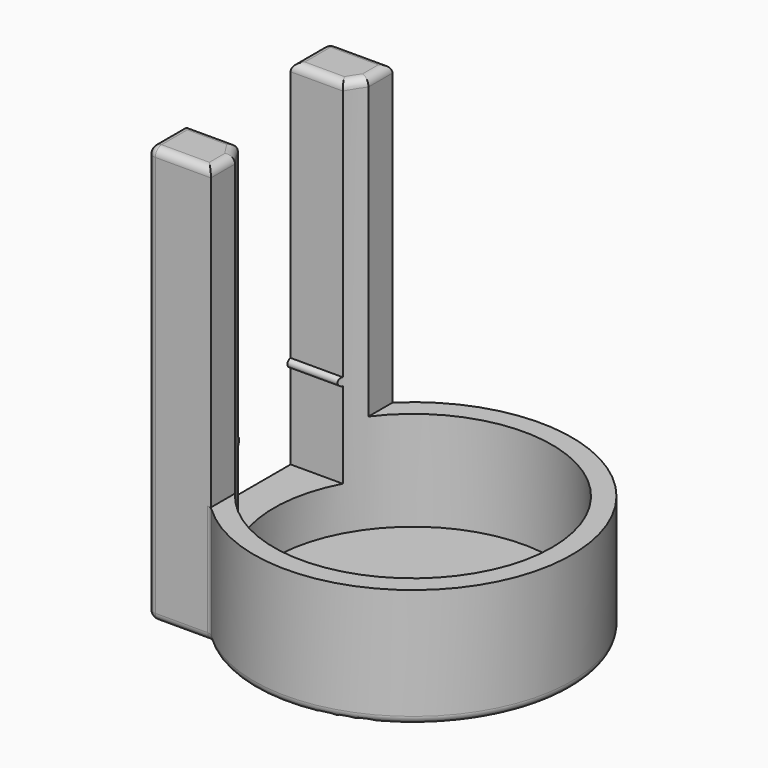
from build123d import *

# Parameters (mm, degrees)
F0_R      = 20
F1_DEPTH  = 50
F2_DEPTH  = 2.5
F4_W      = 40
F4_H      = 50
F5_DEPTH  = 25
F6_W      = 8
F6_H      = 28.5657137142
F7_DEPTH  = 2.5
F8_DEPTH  = 50
F3_R      = 17.5
F9_DEPTH  = 50
F11_DEPTH = 25
F12_R     = 1


with BuildPart() as f1:
    # F0 (on Top) → F1 (new body)
    with BuildSketch(Plane.XY):
        Circle(F0_R)
    extrude(amount=F1_DEPTH)

    # F2 (add): a face of the model
    f2_faces = [f1.faces().sort_by_distance(p)[0] for p in [
        (0, 0, 0),
    ]]
    extrude(f2_faces, amount=F2_DEPTH)

    # F4 (on Front) → F5 (cut, symmetric)
    with BuildSketch(Plane.XZ):
        with Locations((6, 37.5)):
            Rectangle(F4_W, F4_H)
    extrude(amount=F5_DEPTH, both=True, mode=Mode.SUBTRACT)

    # F6 (on Top) → F7 (join)
    with BuildSketch(Plane.XY):
        with Locations((-18, 0)):
            Rectangle(F6_W, F6_H)
    extrude(amount=-F7_DEPTH)

    # F6 (on Top) → F8 (join)
    with BuildSketch(Plane.XY):
        with Locations((-18, 0)):
            Rectangle(F6_W, F6_H)
    extrude(amount=F8_DEPTH)

    # F3 (on Top) → F9 (cut)
    with BuildSketch(Plane.XY):
        Circle(F3_R)
    extrude(amount=F9_DEPTH, mode=Mode.SUBTRACT)

    # F10 (on Right) → F11 (cut)
    with BuildSketch(Plane.YZ):
        with BuildLine():
            Line((8.25, 17.3), (8.25, 50.5))
            Line((8.25, 50.5), (-8.25, 50.5))
            Line((-8.25, 50.5), (-8.25, 17.3))
            ThreePointArc((-8.25, 17.3), (-7.8964466094, 17.1535533906), (-7.75, 16.8))
            ThreePointArc((-7.75, 16.8), (-7.8964466094, 16.4464466094), (-8.25, 16.3))
            Line((-8.25, 16.3), (-8.25, 5.5))
            Line((-8.25, 5.5), (8.25, 5.5))
            Line((8.25, 5.5), (8.25, 16.3))
            ThreePointArc((8.25, 16.3), (7.75, 16.8), (8.25, 17.3))
        make_face()
    extrude(amount=-F11_DEPTH, mode=Mode.SUBTRACT)

    # F12
    f12_edges = [f1.edges().sort_by_distance(p)[0] for p in [
        (20, 0, -2.5),
        (-18, 14.282857, -2.5),
        (-22, 0, -2.5),
        (-18, -14.282857, -2.5),
        (-14, -14.282857, 5),
        (-14, 14.282857, 5),
        (-22, 14.282857, 23.75),
        (-22, -14.282857, 23.75),
        (-14.759599, -9.402352, 50),
        (-14, -12.391428, 50),
        (-18, -14.282857, 50),
        (-22, -11.266428, 50),
        (-18.716662, -8.25, 50),
        (-14, 12.391428, 50),
        (-14.759599, 9.402352, 50),
        (-18.716662, 8.25, 50),
        (-22, 11.266428, 50),
        (-18, 14.282857, 50),
    ]]
    fillet(f12_edges, radius=F12_R)


solid = f1.part
